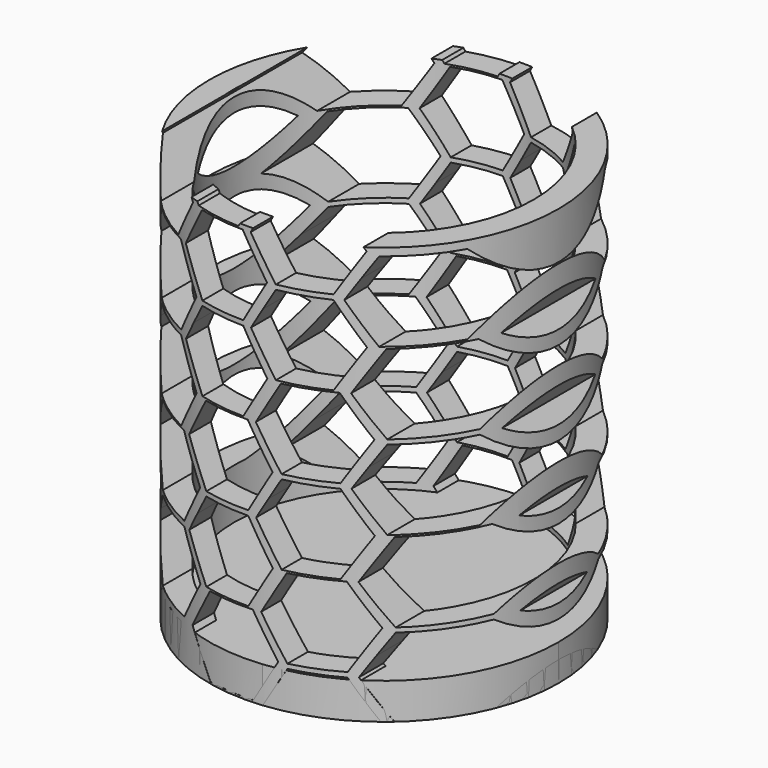
from build123d import *

# Parameters (mm, degrees)
F4_DEPTH = 115.4402024428
F6_DEPTH = 5


with BuildPart() as f1:
    # F0 (on Front) → F1 (revolve)
    with BuildSketch(Plane.XZ):
        Polygon((-43.0947579443, 38.9213711023), (-46.5423390269, 38.9213711023), (-46.5423390269, -18.7802426517), (-22.4031365841, -18.7802426517), (-22.4031365841, -14.4254034385), (-43.0947579443, -14.4254034385), align=None)
    revolve(axis=Axis((-22.4031365841, 0, -16.6028230451), (0, 0, -1)))


with BuildPart() as f1_1:
    # F2: moved
    add(f1.part.moved(Location((1, 91.3, -0.8))))

    # F3 (on Front) → F4 (cut, through all)
    with BuildSketch(Plane.XZ):
        Polygon((-10.9654511504, 32.1066951555), (-9.3964146581, 34.8673939473), (-7.8273781658, 37.6280927392), (-11.0400122453, 43.1064424546), (-17.3907193095, 43.0633945863), (-20.5287922941, 37.5419970027), (-17.3161582145, 32.0636472873), align=None)
        Polygon((43.9869527908, -8.4968721807), (45.5559892831, -5.7361733889), (47.1250257754, -2.975474597), (43.9123916959, 2.5028751184), (37.5616846318, 2.4598272501), (34.4236116472, -3.0615703335), (37.6362457267, -8.5399200489), align=None)
        Polygon((55.1778110199, -14.7760038643), (48.8271039558, -14.8190517325), (45.6890309712, -20.3404493161), (48.9016650507, -25.8187990315), (55.2523721148, -25.7757511633), (56.8214086071, -23.0150523715), (58.3904450994, -20.2543535797), align=None)
        Polygon((65.8304450994, -20.1592163575), (67.3994815917, -17.3985175657), (68.968518084, -14.6378187738), (65.7558840045, -9.1594690584), (59.4051769404, -9.2025169267), (56.2671039558, -14.7239145103), (59.4797380353, -20.2022642257), align=None)
        Polygon((-42.6996701042, 15.257090738), (-41.1306336119, 18.0177895299), (-39.5615971196, 20.7784883217), (-42.7742311991, 26.2568380371), (-49.1249382632, 26.2137901689), (-52.2630112478, 20.6923925852), (-49.0503771683, 15.2140428698), align=None)
        Polygon((23.5181531611, -42.6253555808), (25.0871896534, -39.864656789), (26.6562261457, -37.1039579971), (23.4435920661, -31.6256082817), (17.092885002, -31.66865615), (13.9548120174, -37.1900537336), (17.1674460969, -42.668403449), align=None)
        Polygon((32.7215334668, 8.7820068019), (34.2905699591, 11.5427055937), (35.8596064514, 14.3034043856), (32.6469723719, 19.781754101), (26.2962653077, 19.7387062327), (23.1581923231, 14.2173086491), (26.3708264027, 8.7389589337), align=None)
        Polygon((33.3343187113, -3.1136596875), (26.9836116472, -3.1567075557), (23.8455386626, -8.6781051393), (27.0581727421, -14.1564548548), (33.4088798062, -14.1134069865), (34.9779162985, -11.3527081947), (36.5469527908, -8.5920094029), align=None)
        Polygon((37.2342991303, -31.4874231913), (34.0216650507, -26.0090734759), (27.6709579866, -26.0521213441), (24.532885002, -31.5735189278), (27.7455190815, -37.0518686432), (34.0962261457, -37.008820775), (35.665262638, -34.2481219831), align=None)
        Polygon((15.3908068217, -19.8250790145), (12.1781727421, -14.3467292991), (5.827465678, -14.3897771673), (2.6893926934, -19.911174751), (5.9020267729, -25.3895244664), (12.2527338371, -25.3464765982), (13.8217703294, -22.5857778063), align=None)
        Polygon((44.6742991303, -31.3922859691), (46.2433356225, -28.6315871773), (47.8123721148, -25.8708883855), (44.5997380353, -20.3925386701), (38.2490309712, -20.4355865383), (35.1109579866, -25.956984122), (38.3235920661, -31.4353338374), align=None)
        Polygon((1.6746608525, -30.963011404), (3.2436973448, -28.2023126122), (4.8127338371, -25.4416138203), (1.6000997575, -19.9632641049), (-4.7506073066, -20.0063119732), (-7.8886802912, -25.5277095568), (-4.6760462117, -31.0060592722), align=None)
        Polygon((10.8780411582, 20.4443509787), (12.4470776505, 23.2050497705), (14.0161141428, 25.9657485624), (10.8034800633, 31.4440982778), (4.4527729991, 31.4010504095), (1.3147000145, 25.8796528259), (4.5273340941, 20.4013031105), align=None)
        Polygon((-10.3526659059, 20.2110286661), (-16.70337297, 20.1679807979), (-19.8414459546, 14.6465832142), (-16.6288118751, 9.1682334988), (-10.278104811, 9.2112813671), (-8.7090683187, 11.9719801589), (-7.1400318264, 14.7326789507), align=None)
        Polygon((-42.0123237647, -7.6383230504), (-40.4432872724, -4.8776242586), (-38.8742507801, -2.1169254668), (-42.0868848597, 3.3614242487), (-48.4375919238, 3.3183763804), (-51.5756649084, -2.2030212032), (-48.3630308289, -7.6813709186), align=None)
        Polygon((-43.3870164436, 38.1525045265), (-41.8179799513, 40.9132033183), (-40.248943459, 43.6739021101), (-43.4615775385, 49.1522518255), (-49.8122846027, 49.1092039573), (-52.9503575872, 43.5878063736), (-49.7377235077, 38.1094566582), align=None)
        Polygon((-21.543524135, 26.4901603497), (-19.9744876427, 29.2508591415), (-18.4054511504, 32.0115579333), (-21.6180852299, 37.4899076487), (-27.9687922941, 37.4468597805), (-31.1068652786, 31.9254621969), (-27.8942311991, 26.4471124814), align=None)
        Polygon((-20.8561777956, 3.5947465612), (-19.2871413033, 6.3554453531), (-17.718104811, 9.1161441449), (-20.9307388905, 14.5944938603), (-27.2814459546, 14.5514459921), (-30.4195189392, 9.0300484084), (-27.2068848597, 3.551698693), align=None)
        Polygon((-28.2961777956, 3.4996093391), (-31.5088118751, 8.9779590545), (-37.8595189392, 8.9349111862), (-40.9975919238, 3.4135136026), (-37.7849578443, -2.0648361128), (-31.4342507801, -2.0217882446), (-29.8652142878, 0.7389105472), align=None)
        Polygon((22.8308068217, -19.7299417923), (24.3998433139, -16.9692430005), (25.9688798062, -14.2085442087), (22.7562457267, -8.7301944933), (16.4055386626, -8.7732423615), (13.267465678, -14.2946399452), (16.4800997575, -19.7729896606), align=None)
        Polygon((22.1434604822, 3.1654719961), (23.7124969745, 5.9261707879), (25.2815334668, 8.6868695797), (22.0688993873, 14.1652192952), (15.7181923231, 14.1221714269), (12.5801193386, 8.6007738433), (15.7927534181, 3.1224241279), align=None)
        Polygon((-32.808943459, 43.7690393323), (-31.2399069667, 46.5297381241), (-29.6708704744, 49.2904369159), (-32.8835045539, 54.7687866314), (-39.2342116181, 54.7257387631), (-42.3722846027, 49.2043411795), (-39.1596505231, 43.7259914641), align=None)
        Polygon((54.5650257754, -2.8803373749), (56.1340622677, -0.119638583), (57.70309876, 2.6410602088), (54.4904646805, 8.1194099242), (48.1397576163, 8.0763620559), (45.0016846318, 2.5549644723), (48.2143187113, -2.9233852431), align=None)
        Polygon((0.2999681736, 14.8278161729), (1.8690046659, 17.5885149647), (3.4380411582, 20.3492137565), (0.2254070787, 25.8275634719), (-6.1252999855, 25.7845156037), (-9.26337297, 20.2631180201), (-6.0507388905, 14.7847683047), align=None)
        Polygon((-32.1961582145, 31.8733728429), (-38.5468652786, 31.8303249747), (-41.6849382632, 26.308927391), (-38.4723041837, 20.8305776756), (-32.1215971196, 20.8736255439), (-30.5525606273, 23.6343243357), (-28.983524135, 26.3950231275), align=None)
        Polygon((-6.452685487, -8.1627348377), (-9.6653195665, -2.6843851223), (-16.0160266306, -2.7274329906), (-19.1540996152, -8.2488305742), (-15.9414655357, -13.7271802896), (-9.5907584715, -13.6841324214), (-8.0217219792, -10.9234336295), align=None)
        Polygon((27.0583615199, -14.786058412), (25.4529793537, -17.5677903258), (23.8839012931, -20.2866161657), (27.0602939293, -25.7860582423), (33.4111467924, -25.7849425652), (36.5856070192, -20.2843848115), (33.409214383, -14.7849427349), align=None)
        Polygon((76.408518084, -14.5426815517), (77.9775545763, -11.7819827598), (79.5465910686, -9.021283968), (76.3339569891, -3.5429342526), (69.9832499249, -3.5859821208), (66.8451769404, -9.1073797045), (70.0578110199, -14.5857294199), align=None)
        Polygon((27.7457078593, -37.6814722004), (26.1403256931, -40.4632041142), (24.5712476325, -43.1820299541), (27.7476402687, -48.6814720307), (34.0984931318, -48.6803563536), (37.2729533587, -43.1797986), (34.0965607224, -37.6803565234), align=None)
        Polygon((-39.1594617453, 43.0963879068), (-40.7648439116, 40.314655993), (-42.3339219722, 37.5958301532), (-39.1575293359, 32.0963880766), (-32.8066764729, 32.0975037536), (-29.632216246, 37.5980615073), (-32.8086088822, 43.0975035839), align=None)
        Polygon((-64.5431624128, 26.9194349148), (-62.9741259205, 29.6801337067), (-61.4050894282, 32.4408324985), (-64.6177235077, 37.9191822139), (-70.9684305718, 37.8761343456), (-74.1065035564, 32.354736762), (-70.8938694769, 26.8763870466), align=None)
        Polygon((0.987314513, -8.0675976155), (2.5563510053, -5.3068988237), (4.1253874976, -2.5462000319), (0.9127534181, 2.9321496835), (-5.437953646, 2.8891018153), (-8.5760266306, -2.6322957684), (-5.3633925511, -8.1106454838), align=None)
        Polygon((-53.9650894282, 32.5359697207), (-52.3960529359, 35.2966685125), (-50.8270164436, 38.0573673043), (-54.0396505231, 43.5357170197), (-60.3903575872, 43.4926691515), (-63.5284305718, 37.9712715678), (-60.3157964923, 32.4929218524), align=None)
        Polygon((-60.3156077145, 31.8633182952), (-61.9209898807, 29.0815863814), (-63.4900679414, 26.3627605415), (-60.3136753051, 20.8633184649), (-53.962822442, 20.864434142), (-50.7883622152, 26.3649918957), (-53.9647548514, 31.8644339723), align=None)
        Polygon((26.3710151805, 8.1093553764), (24.7656330143, 5.3276234627), (23.1965549536, 2.6087976228), (26.3729475899, -2.8906444538), (32.7238004529, -2.8895287767), (35.8982606798, 2.6110289769), (32.7218680436, 8.1104710535), align=None)
        Polygon((58.7925804737, 2.0635460055), (57.1871983074, -0.7181859083), (55.6181202468, -3.4370117482), (58.7945128831, -8.9364538248), (65.1453657461, -8.9353381477), (68.319825973, -3.434780394), (65.1434333368, 2.0646616825), align=None)
        Polygon((-5.3632037733, -8.740249041), (-6.9685859395, -11.5219809548), (-8.5376640001, -14.2408067947), (-5.3612713639, -19.7402488713), (0.9895814992, -19.7391331942), (4.164041726, -14.2385754405), (0.9876490898, -8.7391333639), align=None)
        Polygon((16.4802885353, -20.4025932178), (14.8749063691, -23.1843251316), (13.3058283085, -25.9031509715), (16.4822209447, -31.4025930481), (22.8330738078, -31.401477371), (26.0075340346, -25.9009196173), (22.8311413984, -20.4014775407), align=None)
        Polygon((-15.9412767579, -14.3567838468), (-17.5466589241, -17.1385157606), (-19.1157369847, -19.8573416005), (-15.9393443485, -25.3567836771), (-9.5884914854, -25.355668), (-6.4140312585, -19.8551102464), (-9.5904238948, -14.3556681698), align=None)
        Polygon((15.7929421959, 2.4928205706), (14.1875600297, -0.2889113432), (12.618481969, -3.007737183), (15.7948746053, -8.5071792596), (22.1457274684, -8.5060635826), (25.3201876952, -3.0055058289), (22.143795059, 2.4939362477), align=None)
        Polygon((-50.1396701042, 15.1619535159), (-53.3523041837, 20.6403032313), (-59.7030112478, 20.597255363), (-62.8410842324, 15.0758577794), (-59.6284501529, 9.597508064), (-53.2777430887, 9.6405559322), (-51.7087065965, 12.401254724), align=None)
        Polygon((-75.1212353973, 21.302900109), (-73.5521989051, 24.0635989008), (-71.9831624128, 26.8242976927), (-75.1957964923, 32.3026474081), (-81.5465035564, 32.2595995398), (-84.684576541, 26.7382019562), (-81.4719424615, 21.2598522408), align=None)
        Polygon((-28.5813887607, 48.7129227126), (-30.186770927, 45.9311907989), (-31.7558489876, 43.212364959), (-28.5794563514, 37.7129228824), (-22.2286034883, 37.7140385595), (-19.0541432614, 43.2145963131), (-22.2305358976, 48.7140383897), align=None)
        Polygon((5.2148692113, -3.1237142352), (3.6094870451, -5.905446149), (2.0404089845, -8.6242719889), (5.2168016207, -14.1237140655), (11.5676544838, -14.1225983884), (14.7421147106, -8.6220406347), (11.5657220744, -3.1225985581), align=None)
        Polygon((-37.7847690665, -2.69443967), (-39.3901512327, -5.4761715838), (-40.9592292933, -8.1949974237), (-37.7828366571, -13.6944395003), (-31.431983794, -13.6933238232), (-28.2575235672, -8.1927660696), (-31.4339162034, -2.693323993), align=None)
        Polygon((36.9490881651, 13.7258901823), (35.3437059988, 10.9441582685), (33.7746279382, 8.2253324286), (36.9510205744, 2.725890352), (43.3018734375, 2.7270060291), (46.4763336644, 8.2275637827), (43.2999410282, 13.7270058593), align=None)
        Polygon((37.6364345045, -9.1695236062), (36.0310523383, -11.95125552), (34.4619742776, -14.6700813598), (37.6383669139, -20.1695234364), (43.989219777, -20.1684077594), (47.1636800038, -14.6678500057), (43.9872873676, -9.1684079291), align=None)
        Polygon((-6.7378964521, 37.0505785359), (-8.3432786184, 34.2688466221), (-9.912356679, 31.5500207822), (-6.7359640428, 26.0505787056), (-0.3851111797, 26.0516943827), (2.7893490472, 31.5522521363), (-0.387043589, 37.0516942129), align=None)
        Polygon((-70.8936806991, 26.2467834894), (-72.4990628653, 23.4650515756), (-74.0681409259, 20.7462257357), (-70.8917482897, 15.2467836591), (-64.5408954266, 15.2478993362), (-61.3664351998, 20.7484570898), (-64.542827836, 26.2478991664), align=None)
        Polygon((-49.7375347299, 37.479853101), (-51.3429168961, 34.6981211872), (-52.9119949568, 31.9792953473), (-49.7356023205, 26.4798532707), (-43.3847494574, 26.4809689478), (-40.2102892306, 31.9815267015), (-43.3866818668, 37.4809687781), align=None)
        Polygon((48.2145074891, -3.5529888003), (46.6091253229, -6.3347207141), (45.0400472622, -9.053546554), (48.2164398985, -14.5529886306), (54.5672927615, -14.5518729535), (57.7417529884, -9.0513151999), (54.5653603522, -3.5518731233), align=None)
        Polygon((-17.3159694367, 31.43404373), (-18.921351603, 28.6523118162), (-20.4904296636, 25.9334859764), (-17.3140370273, 20.4340438998), (-10.9631841643, 20.4351595768), (-7.7887239374, 25.9357173305), (-10.9651165736, 31.4351594071), align=None)
        Polygon((5.9022155507, -26.0191280236), (4.2968333845, -28.8008599374), (2.7277553239, -31.5196857773), (5.9041479601, -37.0191278539), (12.2550008232, -37.0180121768), (15.4294610501, -31.5174544232), (12.2530684138, -26.0180123466), align=None)
        Polygon((-59.6282613751, 8.9679045067), (-61.2336435413, 6.186172593), (-62.8027216019, 3.4673467531), (-59.6263289657, -2.0320953235), (-53.2754761026, -2.0309796465), (-50.1010158758, 3.4695781072), (-53.277408512, 8.9690201838), align=None)
        Polygon((-81.4717536837, 20.6302486835), (-83.0771358499, 17.8485167698), (-84.6462139105, 15.1296909299), (-81.4698212743, 9.6302488533), (-75.1189684112, 9.6313645303), (-71.9445081844, 15.131922284), (-75.1209008206, 20.6313643606), align=None)
        Polygon((-63.8558160733, 4.0240211264), (-62.286779581, 6.7847199182), (-60.7177430887, 9.54541871), (-63.9303771683, 15.0237684254), (-70.2810842324, 14.9807205572), (-73.419157217, 9.4593229736), (-70.2065231375, 3.9809732582), align=None)
        Polygon((80.6360727823, -9.5987981713), (79.030690616, -12.3805300851), (77.4616125554, -15.099355925), (80.6380051917, -20.5987980016), (86.9888580547, -20.5976823245), (90.1633182816, -15.0971245708), (86.9869256454, -9.5976824942), align=None)
        Polygon((-84.1302718896, 18.447064095), (-82.5612353973, 21.2077628868), (-85.7738694769, 26.6861126022), (-92.124576541, 26.643064734), (-95.2626495256, 21.1216671504), (-92.0500154461, 15.6433174349), (-85.6993083819, 15.6863653032), align=None)
        Polygon((-20.1688314561, -19.3006672272), (-18.5997949638, -16.5399684354), (-17.0307584715, -13.7792696435), (-20.2433925511, -8.3009199281), (-26.5940996152, -8.3439677964), (-29.7321725998, -13.86536538), (-26.5195385203, -19.3437150954), align=None)
        Polygon((11.4908264027, 8.5486844893), (5.1401193386, 8.5056366211), (2.002046354, 2.9842390374), (5.2146804335, -2.494110678), (11.5653874976, -2.4510628097), (13.1344239899, 0.3096359821), (14.7034604822, 3.0703347739), align=None)
        Polygon((-38.4721154059, 20.2009741184), (-40.0774975721, 17.4192422046), (-41.6465756328, 14.7004163647), (-38.4701829965, 9.2009742881), (-32.1193301334, 9.2020899652), (-28.9448699066, 14.7026477189), (-32.1212625428, 20.2020897955), align=None)
        Polygon((59.4799268131, -20.831867783), (57.8745446469, -23.6135996967), (56.3054665862, -26.3324255366), (59.4818592225, -31.8318676132), (65.8327120856, -31.8307519362), (69.0071723124, -26.3301941825), (65.8307796762, -20.8307521059), align=None)
        Polygon((-27.8940424213, 25.8175089242), (-29.4994245875, 23.0357770104), (-31.0685026482, 20.3169511705), (-27.8921100119, 14.8175090939), (-21.5412571488, 14.818624771), (-18.366796922, 20.3191825247), (-21.5431895582, 25.8186246013), align=None)
        Polygon((-49.0501883905, 14.5844393126), (-50.6555705567, 11.8027073988), (-52.2246486173, 9.0838815589), (-49.0482559811, 3.5844394823), (-42.697403118, 3.5855551594), (-39.5229428912, 9.086112913), (-42.6993355274, 14.5855549896), align=None)
        Polygon((-27.2066960819, 2.9220951358), (-28.8120782481, 0.140363222), (-30.3811563087, -2.5784626179), (-27.2047636725, -8.0779046945), (-20.8539108094, -8.0767890174), (-17.6794505826, -2.5762312638), (-20.8558432188, 2.9232108128), align=None)
        Polygon((15.1055958565, 25.3882343591), (13.5002136902, 22.6065024453), (11.9311356296, 19.8876766054), (15.1075282658, 14.3882345288), (21.4583811289, 14.3893502059), (24.6328413558, 19.8899079595), (21.4564487196, 25.3893500361), align=None)
        Polygon((4.5275228719, 19.7716995532), (2.9221407057, 16.9899676395), (1.353062645, 14.2711417996), (4.5294552813, 8.771699723), (10.8803081443, 8.7728154), (14.0547683712, 14.2733731537), (10.878375735, 19.7728152303), align=None)
        Polygon((48.9018538285, -26.4484025888), (47.2964716623, -29.2301345026), (45.7273936017, -31.9489603424), (48.9037862379, -37.448402419), (55.254639101, -37.447286742), (58.4290993278, -31.9467289883), (55.2527066916, -26.4472869117), align=None)
        Polygon((-6.0505501127, 14.1551647474), (-7.6559322789, 11.3734328336), (-9.2250103396, 8.6546069938), (-6.0486177033, 3.1551649172), (0.3022351598, 3.1562805942), (3.4766953866, 8.6568383479), (0.3003027504, 14.1562804245), align=None)
        Polygon((-16.6286230973, 8.5386299416), (-18.2340052635, 5.7568980278), (-19.8030833242, 3.0380721879), (-16.6266906879, -2.4613698887), (-10.2758378248, -2.4602542116), (-7.101377598, 3.0403035421), (-10.2777702342, 8.5397456187), align=None)
        Polygon((70.0579997977, -15.2153329771), (68.4526176315, -17.9970648909), (66.8835395708, -20.7158907308), (70.0599322071, -26.2153328074), (76.4107850702, -26.2142171303), (79.585245297, -20.7136593767), (76.4088526608, -15.2142173001), align=None)
        Polygon((38.3237808439, -32.0649373946), (36.7183986777, -34.8466693084), (35.1493206171, -37.5654951483), (38.3257132533, -43.0649372249), (44.6765661164, -43.0638215478), (47.8510263432, -37.5632637941), (44.674633707, -32.0638217175), align=None)
    extrude(amount=-F4_DEPTH, mode=Mode.SUBTRACT)


with BuildPart() as f6:
    # F5 (on face) → F6 (new body)
    with BuildSketch(Plane(origin=(0, 0, -19.5802426517), x_dir=(1, 0, 0), z_dir=(0, 0, -1))):
        with BuildLine():
            ThreePointArc((-18.9558187307, -115.3148231287), (-3.4897701266, -107.4806179343), (2.7360658587, -91.3))
            ThreePointArc((2.7360658587, -91.3), (-3.4897701266, -75.1193820657), (-18.9558187307, -67.2851768713))
            Line((-18.9558187307, -67.2851768713), (-18.9558187307, -115.3148231287))
        make_face()
        with BuildLine():
            Line((-18.9558187307, -115.3148231287), (-18.9558187307, -67.2851768713))
            ThreePointArc((-18.9558187307, -67.2851768713), (-37.5837545184, -73.3866335425), (-45.5423390269, -91.3))
            ThreePointArc((-45.5423390269, -91.3), (-37.5837545184, -109.2133664575), (-18.9558187307, -115.3148231287))
        make_face()
    extrude(amount=-F6_DEPTH)


solid = Compound([f1_1.part, f6.part])
